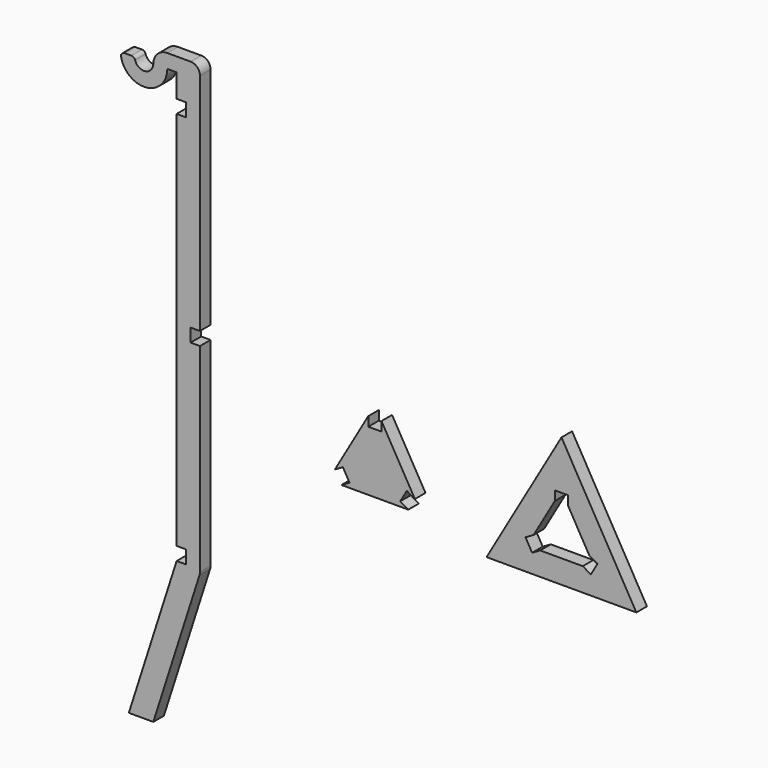
from build123d import *

# Parameters (mm, degrees)
F1_W     = 12.7
F1_H     = 19.05
F2_DEPTH = 18.034
F3_R     = 12.7
F4_R     = 5.08


# Not quite as in the source:
# - a variable given as a bare number and used for a length is read in inches; the dataset says mm whatever the document's units were


with BuildPart() as f2:
    # F1 (on Front) → F2 (new body)
    with BuildSketch(Plane.XZ):
        Polygon((15.875, 403.91953125), (-15.875, 403.91953125), (-15.875, 384.86953125), (-15.875, 353.11953125), (-3.175, 353.11953125), (-3.175, 335.08553125), (-15.875, 335.08553125), (-15.875, -182.68553125), (-3.175, -182.68553125), (-3.175, -200.71953125), (-15.875, -200.71953125), (-80.9640890891, -403.91953125), (-47.625, -403.91953125), (15.875, -205.68046875), (15.875, 67.183), (3.175, 67.183), (3.175, 76.2), (3.175, 85.217), (15.875, 85.217), align=None)
        with BuildLine():
            ThreePointArc((-92.075, 384.86953125), (-60.325, 353.11953125), (-28.575, 384.86953125))
            Line((-28.575, 384.86953125), (-47.625, 384.86953125))
            ThreePointArc((-47.625, 384.86953125), (-60.325, 372.16953125), (-73.025, 384.86953125))
            Line((-73.025, 384.86953125), (-92.075, 384.86953125))
        make_face()
        with BuildLine():
            Line((-28.575, 384.86953125), (-28.575, 403.91953125))
            ThreePointArc((-28.575, 403.91953125), (-42.0453841816, 398.3399154316), (-47.625, 384.86953125))
            Line((-47.625, 384.86953125), (-28.575, 384.86953125))
        make_face()
        with Locations((-22.225, 394.39453125)):
            Rectangle(F1_W, F1_H)
    extrude(amount=F2_DEPTH)

    # F3
    f3_edges = [f2.edges().sort_by_distance(p)[0] for p in [
        (15.875, -9.017, -205.680469),
        (15.875, -9.017, 403.919531),
    ]]
    fillet(f3_edges, radius=F3_R)

    # F4
    f4_edges = [f2.edges().sort_by_distance(p)[0] for p in [
        (-73.025, -9.017, 384.869531),
        (-92.075, -9.017, 384.869531),
    ]]
    fillet(f4_edges, radius=F4_R)


with BuildPart() as f2b:
    # F1 (on Front) → F2, piece 2 (new body)
    with BuildSketch(Plane.XZ):
        Polygon((208.534, -36.6617420935), (299.466, -36.6617420935), (288.4674773719, -30.3117420935), (297.4844773719, -14.6938399617), (308.483, -21.0438399617), (263.017, 57.7055820552), (263.017, 45.0055820552), (244.983, 45.0055820552), (244.983, 57.7055820552), (199.517, -21.0438399617), (210.5155226281, -14.6938399617), (219.5325226281, -30.3117420935), align=None)
    extrude(amount=F2_DEPTH)


with BuildPart() as f2c:
    # F1 (on Front) → F2, piece 3 (new body)
    with BuildSketch(Plane.XZ):
        Polygon((406.0051708018, -58.8867420935), (609.9948291982, -58.8867420935), (508, 117.7734841871), align=None)
        Polygon((470.0147839421, -11.5188399617), (498.983, 38.6555820552), (498.983, 51.3555820552), (517.017, 51.3555820552), (517.017, 38.6555820552), (545.9852160579, -11.5188399617), (556.983738686, -17.8688399617), (547.966738686, -33.4867420935), (536.9682160579, -27.1367420935), (479.0317839421, -27.1367420935), (468.033261314, -33.4867420935), (459.016261314, -17.8688399617), align=None, mode=Mode.SUBTRACT)
    extrude(amount=F2_DEPTH)


solid = Compound([f2.part, f2b.part, f2c.part])
